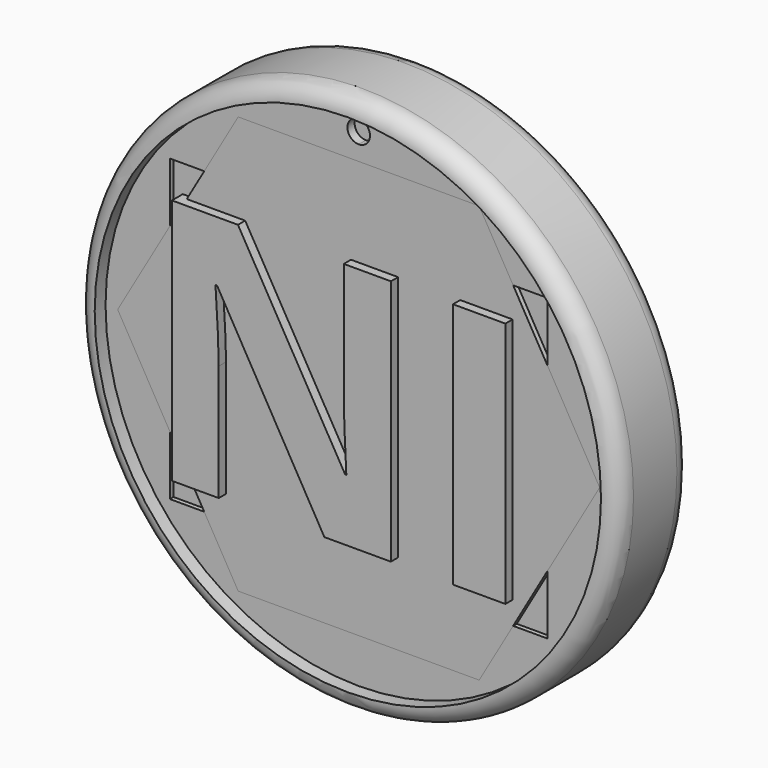
from build123d import *

# Parameters (mm, degrees)
F0_R         = 76.2
F1_DEPTH     = 25.4
F2_R         = 5.08
F3_DEPTH     = 6.35
F5_TEXT_SIZE = 97.1383725603
F8_DEPTH     = 5.08
F7_R         = 71.12
F9_DEPTH     = 2.54
F7_W         = 106.0970500112
F7_H         = 84.2363908887
F10_DEPTH    = 1.27
F11_R        = 5.1309176721
F11_R_2      = 4.9464726209
F11_R_3      = 4.7280466605
F11_R_4      = 5.3151392108
F12_DEPTH    = 6.35
F13_DEPTH    = 2.54


# Not quite as in the source:
# - Text() gives the source's letters only with a copy of the font that has no kerning and outlines rounded to 1/6400 em; it was checked with that copy


with BuildPart() as f1:
    # F0 (on Front) → F1 (new body)
    with BuildSketch(Plane.XZ):
        Circle(F0_R)
    extrude(amount=F1_DEPTH)

    # F2
    f2_edges = [f1.edges().sort_by_distance(p)[0] for p in [
        (-76.2, -25.4, 0),
        (76.2, -12.7, 0),
        (-76.2, 0, 0),
    ]]
    fillet(f2_edges, radius=F2_R)

    # F3 (cut): a face of the model
    f3_faces = [f1.faces().sort_by_distance(p)[0] for p in [
        (0, -25.4, 0),
    ]]
    extrude(f3_faces, amount=-F3_DEPTH, mode=Mode.SUBTRACT)

    # F7 (on face) → F9 (join)
    with BuildSketch(Plane.XZ.offset(19.05)):
        Circle(F7_R)
        Polygon((-53.0485250056, -42.1181954443), (-53.0485250056, 42.1181954443), (0, 42.1181954443), (53.0485250056, 42.1181954443), (53.0485250056, -42.1181954443), align=None, mode=Mode.SUBTRACT)
        with BuildLine():
            ThreePointArc((3.175, 66.04), (2.2450640303, 63.7949359697), (0, 62.865))
            ThreePointArc((0, 62.865), (-2.2450640303, 68.2850640303), (3.175, 66.04))
        make_face(mode=Mode.SUBTRACT)
    extrude(amount=F9_DEPTH)

    # F7 (on face) → F10 (join)
    with BuildSketch(Plane.XZ.offset(19.05)):
        Rectangle(F7_W, F7_H)
    extrude(amount=F10_DEPTH)

    # F11 (on face) → F12 (cut)
    with BuildSketch(Plane.XZ.offset(19.05)):
        with Locations((0, 50.3199957311)):
            Circle(F11_R)
        with Locations((-59.721197933, 0)):
            Circle(F11_R_2)
        with Locations((59.2105202377, 0)):
            Circle(F11_R_3)
        with Locations((0, -51.9960708916)):
            Circle(F11_R_4)
    extrude(amount=F12_DEPTH, mode=Mode.SUBTRACT)


with BuildPart() as f8:
    # F5 (on face) → F8 (new body)
    with BuildSketch(Plane.XZ.offset(19.05)):
        with Locations((-59.1634994489, -35.7186351903)):
            Text('NI', F5_TEXT_SIZE, font='Open Sans', font_style=FontStyle.BOLD, text_align=(TextAlign.LEFT, TextAlign.BOTTOM))
    extrude(amount=F8_DEPTH)


with BuildPart() as f13:
    # F6 (on face) → F13 (new body)
    with BuildSketch(Plane.XZ.offset(19.05)):
        Polygon((33.85394614, 58.6367547512), (-33.85394614, 58.6367547512), (-67.70789228, 0), (-33.85394614, -58.6367547512), (33.85394614, -58.6367547512), (67.70789228, 0), align=None)
    extrude(amount=F13_DEPTH)


solid = Compound([f1.part, f8.part, f13.part])
